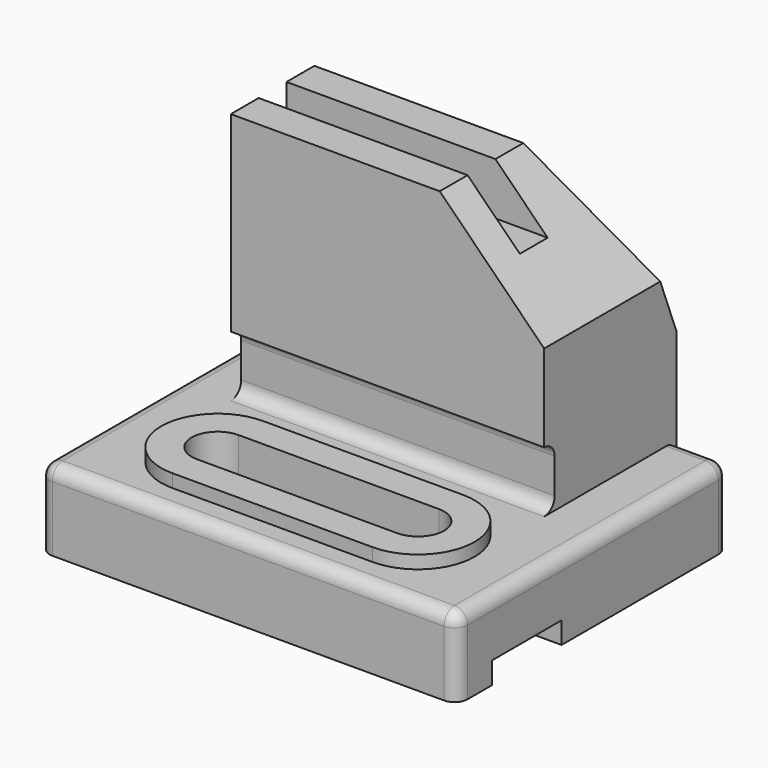
from build123d import *

# Parameters (mm, degrees)
F0_W      = 96
F0_H      = 78
F1_DEPTH  = 18
F2_W      = 72
F2_H      = 38
F4_DEPTH  = 58
F6_DEPTH  = 38
F8_DEPTH  = 72.001
F9_W      = 8
F9_H      = 12
F10_DEPTH = 60.001
F12_DEPTH = 3
F14_DEPTH = 21
F15_W     = 20
F15_H     = 5
F16_DEPTH = 96.001
F17_W     = 3
F17_H     = 14
F18_DEPTH = 72
F19_R     = 2.99999


# Not quite as in the source:
# - a fillet or chamfer is up to 0.001 mm smaller than in the source, because OpenCascade refuses the exact size


with BuildPart() as f1:
    # F0 (on Top) → F1 (new body)
    with BuildSketch(Plane.XY):
        with Locations((48, 39)):
            Rectangle(F0_W, F0_H)
    extrude(amount=F1_DEPTH)

    # F2 (on face) → F4 (join, through all)
    with BuildSketch(Plane.XY.offset(18)):
        with Locations((48, 59)):
            Rectangle(F2_W, F2_H)
    extrude(amount=F4_DEPTH)

    # F5 (on face) → F6 (cut, through all)
    with BuildSketch(Plane.XZ.offset(-40)):
        Polygon((84, 76), (60, 76), (84, 52), align=None)
    extrude(amount=-F6_DEPTH, mode=Mode.SUBTRACT)

    # F7 (on face) → F8 (cut, through all)
    with BuildSketch(Plane(origin=(12, 0, 0), x_dir=(0, -1, 0), z_dir=(-1, 0, 0))):
        Polygon((-78, 76), (-78, 40), (-64, 76), align=None)
    extrude(amount=-F8_DEPTH, mode=Mode.SUBTRACT)

    # F9 (on face) → F10 (cut, through all)
    with BuildSketch(Plane(origin=(12, 0, 0), x_dir=(0, -1, 0), z_dir=(-1, 0, 0))):
        with Locations((-52, 70)):
            Rectangle(F9_W, F9_H)
    extrude(amount=-F10_DEPTH, mode=Mode.SUBTRACT)

    # F11 (on face) → F12 (join)
    with BuildSketch(Plane.XY.offset(18)):
        with BuildLine():
            Line((71, 33), (25, 33))
            ThreePointArc((25, 33), (12, 20), (25, 7))
            Line((25, 7), (71, 7))
            ThreePointArc((71, 7), (84, 20), (71, 33))
        make_face()
    extrude(amount=F12_DEPTH)

    # F13 (on face) → F14 (cut, through all)
    with BuildSketch(Plane.XY.offset(21)):
        with BuildLine():
            Line((71, 26), (25, 26))
            ThreePointArc((25, 26), (19, 20), (25, 14))
            Line((25, 14), (71, 14))
            ThreePointArc((71, 14), (77, 20), (71, 26))
        make_face()
    extrude(amount=-F14_DEPTH, mode=Mode.SUBTRACT)

    # F15 (on face) → F16 (cut, through all)
    with BuildSketch(Plane.YZ.offset(96)):
        with Locations((20, 2.5)):
            Rectangle(F15_W, F15_H)
    extrude(amount=-F16_DEPTH, mode=Mode.SUBTRACT)

    # F17 (on face) → F18 (cut, through all)
    with BuildSketch(Plane.YZ.offset(84)):
        with Locations((41.5, 25)):
            Rectangle(F17_W, F17_H)
    extrude(amount=-F18_DEPTH, mode=Mode.SUBTRACT)

    # F19 (radius 3 in the source; OpenCascade refuses exactly that, so slightly less here)
    f19_edges = [f1.edges().sort_by_distance(p)[0] for p in [
        (48, 43, 18),
        (48, 43, 32),
        (96, 39, 18),
        (48, 0, 18),
        (96, 0, 9),
        (96, 78, 9),
        (90, 78, 18),
        (0, 39, 18),
        (0, 0, 9),
        (0, 78, 9),
        (6, 78, 18),
    ]]
    fillet(f19_edges, radius=F19_R)


solid = f1.part
